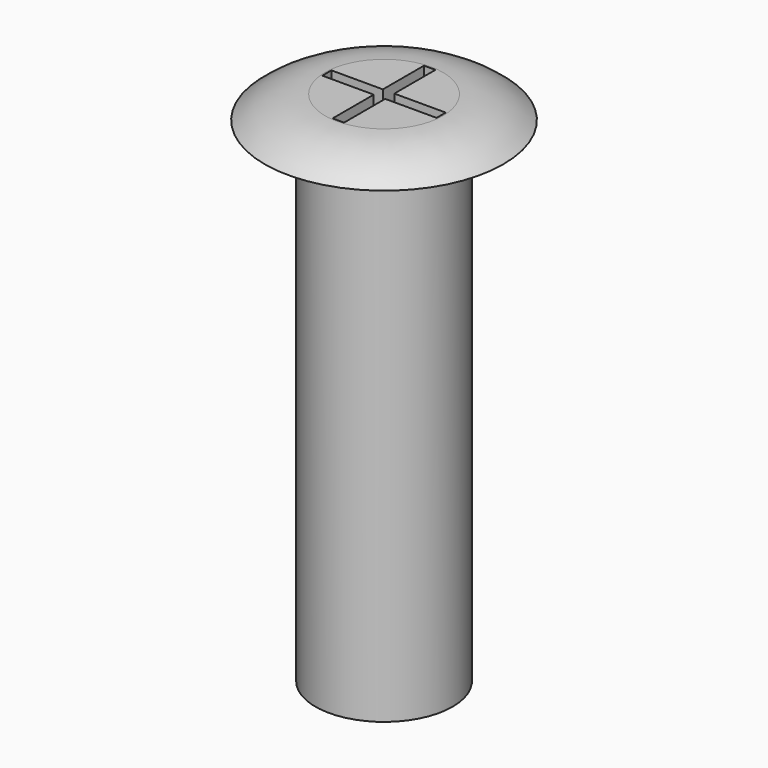
from build123d import *

# Parameters (mm, degrees)
F0_R     = 1.5
F1_DEPTH = 11.3
F2_R     = 2.61
F2_R_2   = 1.5
F3_DEPTH = 0.5
F5_DEPTH = 0.5


# Not quite as in the source:
# - a fillet or chamfer that OpenCascade refuses, or shapes differently, is made with other operations: its cross-section is extruded or revolved along the edge and cut away or added


with BuildPart() as f1:
    # F0 (on Top) → F1 (new body)
    with BuildSketch(Plane.XY):
        Circle(F0_R)
    extrude(amount=F1_DEPTH)

    # F2 (on face) → F3 (join)
    with BuildSketch(Plane.XY.offset(11.3)):
        Circle(F2_R)
        Circle(F2_R_2, mode=Mode.SUBTRACT)
    extrude(amount=-F3_DEPTH)

    # F4: fillet of radius 2 on 1 edges, made by hand

    # F4_s1 → F4_t2 (revolve, cut)
    with BuildSketch(Plane.XZ):
        with BuildLine():
            ThreePointArc((2.61, 10.8), (1.9942311257, 11.1708286934), (1.2871243445, 11.3))
            Line((1.2871243445, 11.3), (2.61, 11.3))
            Line((2.61, 11.3), (2.61, 10.8))
        make_face()
    revolve(axis=Axis((0, 0, 11.3), (0, 0, 1)), mode=Mode.SUBTRACT)

    # F2 (on face) → F5 (cut)
    with BuildSketch(Plane.XY.offset(11.3)):
        Polygon((-1.2485300168, 0.125), (-1.2485300168, -0.125), (-0.125, -0.125), (-0.125, -1.2485300168), (0.125, -1.2485300168), (0.125, -0.125), (1.2485300168, -0.125), (1.2485300168, 0.125), (0.125, 0.125), (0.125, 1.2485300168), (-0.125, 1.2485300168), (-0.125, 0.125), align=None)
    extrude(amount=-F5_DEPTH, mode=Mode.SUBTRACT)


solid = f1.part
